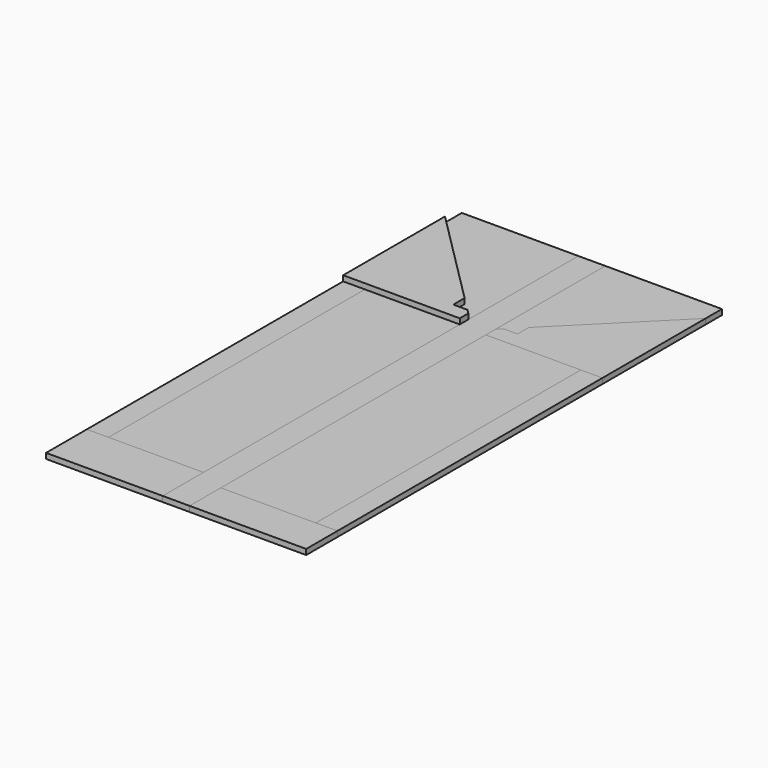
from build123d import *

# Parameters (mm, degrees)
F0_W     = 438
F0_H     = 1478
F1_DEPTH = 25
F0_H_2   = 1528
F2_DEPTH = 25
F0_W_2   = 100
F3_DEPTH = 25
F0_W_3   = 99.9999523163
F4_DEPTH = 25
F5_DEPTH = 25


# Not quite as in the source:
# - ends of sketch curves that miss each other by under 0.0002 mm in the source are joined


with BuildPart() as f1:
    # F0 (on Top) → F1 (new body)
    with BuildSketch(Plane.XY):
        with Locations((319, 974)):
            Rectangle(F0_W, F0_H)
    extrude(amount=F1_DEPTH)


with BuildPart() as f1b:
    # F0 (on Top) → F1, piece 2 (new body)
    with BuildSketch(Plane.XY):
        with Locations((881.0000476837, 944)):
            Rectangle(F0_W, F0_H_2)
    extrude(amount=F1_DEPTH)


with BuildPart() as f2:
    # F0 (on Top) → F2 (new body)
    with BuildSketch(Plane.XY):
        Polygon((682.0000476837, 1785), (662.0000476837, 1765), (662.0000476837, 1708), (1100.0000476837, 1708), (1200.0000476837, 1708), (1200, 2303), (747.0000476837, 1850), (747.0000476837, 1785), align=None)
    extrude(amount=F2_DEPTH)


with BuildPart() as f2b:
    # F0 (on Top) → F2, piece 2 (new body)
    with BuildSketch(Plane.XY):
        Polygon((1100.0000476837, 180), (662.0000476837, 180), (662.0000476837, 0), (1200.0000476837, 0), (1200, 180), align=None)
    extrude(amount=F2_DEPTH)


with BuildPart() as f2c:
    # F0 (on Top) → F2, piece 3 (new body)
    with BuildSketch(Plane.XY):
        Polygon((100, 235), (0, 235), (0, 0), (538, 0), (538, 235), align=None)
    extrude(amount=F2_DEPTH)


with BuildPart() as f2d:
    # F0 (on Top) → F2, piece 4 (new body)
    with BuildSketch(Plane.XY):
        Polygon((453, 1847), (0, 2300), (0, 1713), (100, 1713), (538, 1713), (538, 1762), (518, 1782), (453, 1782), align=None)
    extrude(amount=F2_DEPTH)

    # F0 (on Top) + F2_face (on face) → F4 (join)
    with BuildSketch(Plane.XY):
        Polygon((1200, 2397), (662.0000476837, 2397), (662.0000476837, 1765), (682.0000476837, 1785), (747.0000476837, 1785), (747.0000476837, 1850), (1200.0000476837, 2303), align=None)
        Polygon((538, 2397), (0, 2397), (0, 2300), (453, 1847), (453, 1782), (518, 1782), (538, 1762), align=None)
    with BuildSketch(Plane(origin=(189.6303420005, 1911.2535062619, 25), x_dir=(1, 0, 0), z_dir=(0, 0, 1))):
        Polygon((263.3696579995, -64.2535062619), (-189.6303420005, 388.7464937381), (-189.6303420005, -198.2535062619), (348.3696579995, -198.2535062619), (348.3696579995, -149.2535062619), (328.3696579995, -129.2535062619), (263.3696579995, -129.2535062619), align=None)
    extrude(amount=F4_DEPTH)


with BuildPart() as f3:
    # F0 (on Top) → F3 (new body)
    with BuildSketch(Plane.XY):
        with Locations((50, 974)):
            Rectangle(F0_W_2, F0_H)
    extrude(amount=F3_DEPTH)


with BuildPart() as f3b:
    # F0 (on Top) → F3, piece 2 (new body)
    with BuildSketch(Plane.XY):
        with Locations((1150.0000238419, 944)):
            Rectangle(F0_W_3, F0_H_2)
    extrude(amount=F3_DEPTH)


with BuildPart() as f5:
    # F0 (on Top) → F5 (new body)
    with BuildSketch(Plane.XY):
        Polygon((662.0000476837, 2397), (538, 2397), (538, 1762), (538, 1713), (538, 235), (538, 0), (662.0000476837, 0), (662.0000476837, 180), (662.0000476837, 1708), (662.0000476837, 1765), align=None)
    extrude(amount=F5_DEPTH)


solid = Compound([f1.part, f1b.part, f2.part, f2b.part, f2c.part, f2d.part, f3.part, f3b.part, f5.part])
